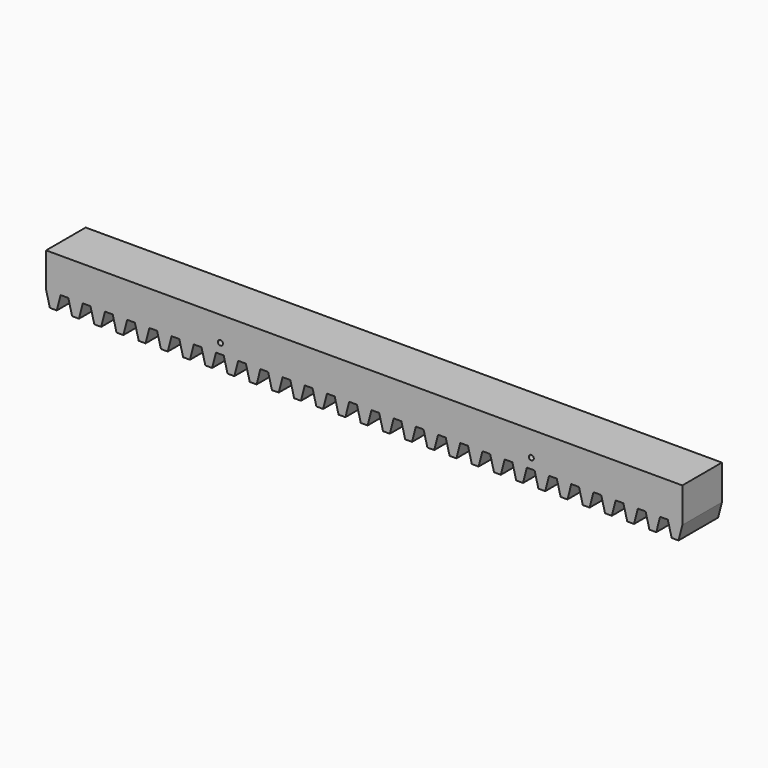
from build123d import *

# Parameters (mm, degrees)
F0_R     = 0.635
F1_DEPTH = 12.7


# Not quite as in the source:
# - a feature of the source that left no trace in its solid (it failed there, or was rolled back) is left out


with BuildPart() as f1:
    # F0 (on Front) → F1 (new body)
    with BuildSketch(Plane.XZ):
        Polygon((26.5642398671, -2.6142263417), (26.5642398671, 6.35), (-136.7738045981, 6.35), (-136.7738045981, -2.5616034378), (-135.7986113058, -6.3323961114), (-134.0326395944, -6.346404838), (-133.0482363701, -2.54), (-131.0740445981, -2.54), (-130.0892531872, -6.3479058444), (-128.3328795944, -6.3651881602), (-127.3484763701, -2.5587833222), (-125.3742845981, -2.5587833222), (-124.3938092991, -6.35), (-122.6284623376, -6.35), (-121.6487163701, -2.5616034378), (-119.6745245981, -2.5616034378), (-118.6947786306, -6.35), (-116.9287023376, -6.35), (-115.9489563701, -2.5616034378), (-113.9747645981, -2.5616034378), (-112.9899731872, -6.3695092822), (-111.2335995944, -6.3680082758), (-110.2491963701, -2.5616034378), (-108.2750045981, -2.5616034378), (-107.2902131872, -6.3695092822), (-105.5338395944, -6.3680082758), (-104.5494363701, -2.5616034378), (-102.5752445981, -2.5616034378), (-101.5904531872, -6.3695092822), (-99.8340795944, -6.3680082758), (-98.8496763701, -2.5616034378), (-96.8754845981, -2.5616034378), (-95.8906931872, -6.3695092822), (-94.1343195944, -6.3680082758), (-93.1499163701, -2.5616034378), (-91.1757245981, -2.5616034378), (-90.1909331872, -6.3695092822), (-88.4345595944, -6.3680082758), (-87.4501563701, -2.5616034378), (-85.4759645981, -2.5616034378), (-84.4911731872, -6.3695092822), (-82.7347995944, -6.386791598), (-81.7503963701, -2.58038676), (-79.7762045981, -2.58038676), (-78.7914131872, -6.3882926044), (-77.0350395944, -6.3680082758), (-76.0506363701, -2.5616034378), (-74.0764445981, -2.5616034378), (-73.0916531872, -6.3695092822), (-71.3352795944, -6.3680082758), (-70.3508763701, -2.5616034378), (-68.3766845981, -2.5616034378), (-67.3918931872, -6.3695092822), (-65.6355195944, -6.3680082758), (-64.6511163701, -2.5616034378), (-62.6769245981, -2.5616034378), (-61.6921331872, -6.3695092822), (-59.9357595944, -6.3680082758), (-58.9513563701, -2.5616034378), (-56.9771645981, -2.5616034378), (-55.9923731872, -6.3695092822), (-54.2264014758, -6.3835180088), (-53.2419982515, -2.5771131708), (-51.2678064795, -2.5771131708), (-50.2830150686, -6.3850190153), (-48.5266414758, -6.402301331), (-47.5422382515, -2.595896493), (-45.5680464795, -2.595896493), (-44.5875711805, -6.3871131708), (-42.822224219, -6.3871131708), (-41.8424782515, -2.5987166086), (-39.8682864795, -2.5987166086), (-38.888540512, -6.3871131708), (-37.122464219, -6.3871131708), (-36.1427182515, -2.5987166086), (-34.1685264795, -2.5987166086), (-33.1837350686, -6.4066224531), (-31.4273614758, -6.4051214466), (-30.4429582515, -2.5987166086), (-28.4687664795, -2.5987166086), (-27.4839750686, -6.4066224531), (-25.7276014758, -6.4051214466), (-24.7431982515, -2.5987166086), (-22.7690064795, -2.5987166086), (-21.7842150686, -6.4066224531), (-20.0278414758, -6.4051214466), (-19.0434382515, -2.5987166086), (-17.0692464795, -2.5987166086), (-16.0844550686, -6.4066224531), (-14.3280814758, -6.4051214466), (-13.3436782515, -2.5987166086), (-11.3694864795, -2.5987166086), (-10.3846950686, -6.4066224531), (-8.6283214758, -6.4051214466), (-7.6439182515, -2.5987166086), (-5.6697264795, -2.5987166086), (-4.6849350686, -6.4066224531), (-2.9285614758, -6.4239047688), (-1.9441582515, -2.6174999308), (0.0300335205, -2.6174999308), (1.0148249314, -6.4254057753), (2.7711985242, -6.4051214466), (3.7556017485, -2.5987166086), (5.7297935205, -2.5987166086), (6.7145849314, -6.4066224531), (8.4709585242, -6.4051214466), (9.4553617485, -2.5987166086), (11.4295535205, -2.5987166086), (12.4143449314, -6.4066224531), (14.1707185242, -6.4051214466), (15.1551217485, -2.5987166086), (17.1293135205, -2.5987166086), (18.1141049314, -6.4066224531), (19.8704785242, -6.4051214466), (20.8548817485, -2.5987166086), (22.8290735205, -2.5987166086), (23.8138649314, -6.4066224531), (25.5798366429, -6.4206311797), align=None)
        with Locations((-92.0139178634, 0.0037964069)):
            Circle(F0_R, mode=Mode.SUBTRACT)
        with Locations((-12.2076766565, 0.0037964069)):
            Circle(F0_R, mode=Mode.SUBTRACT)
    extrude(amount=-F1_DEPTH)


solid = f1.part
